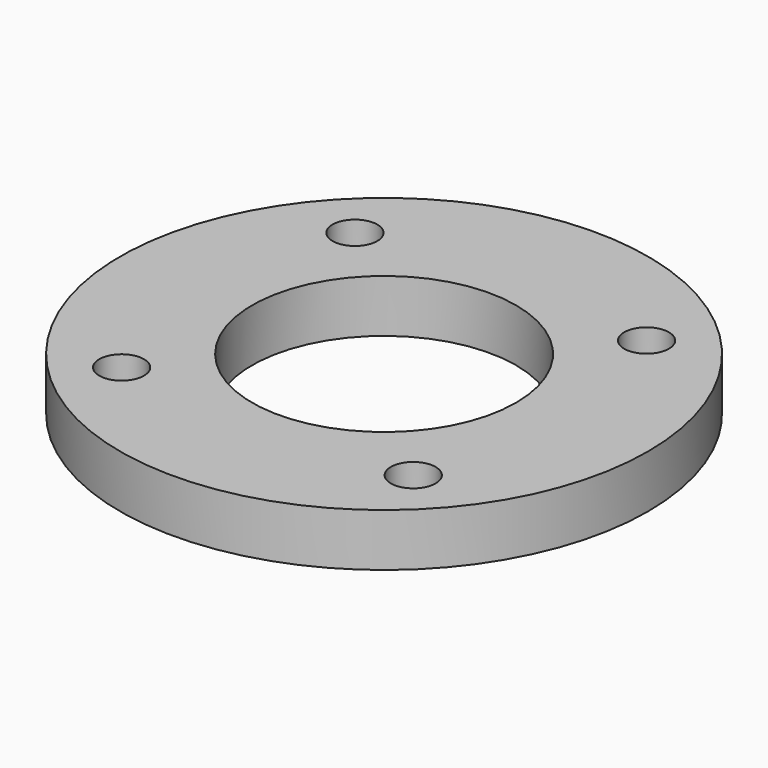
from build123d import *

# Parameters (mm, degrees)
F0_R     = 25.4
F0_R_2   = 2.15265
F0_R_3   = 12.7
F1_DEPTH = 5.08


# Not quite as in the source:
# - a feature names something its author has since deleted; it is built from what else it names


with BuildPart() as f1:
    # F0 (on Top) → F1 (new body)
    with BuildSketch(Plane.XY):
        Circle(F0_R)
        with Locations((-14.0316501892, -14.0316501892)):
            Circle(F0_R_2, mode=Mode.SUBTRACT)
        Circle(F0_R_3, mode=Mode.SUBTRACT)
        with Locations((14.0316501892, -14.0316501892)):
            Circle(F0_R_2, mode=Mode.SUBTRACT)
        with Locations((-14.0316501892, 14.0316501892)):
            Circle(F0_R_2, mode=Mode.SUBTRACT)
        with Locations((14.0316501892, 14.0316501892)):
            Circle(F0_R_2, mode=Mode.SUBTRACT)
    extrude(amount=F1_DEPTH)


solid = f1.part
